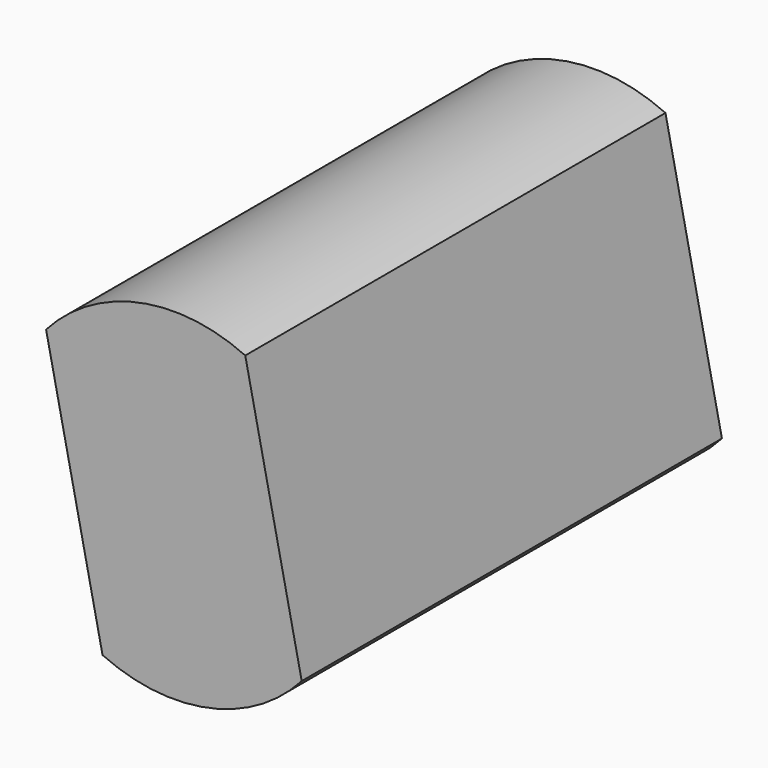
from build123d import *

# Parameters (mm, degrees)
F2_DEPTH = 8


# Not quite as in the source:
# - the program builds the solid bodies; features that only make, move or delete a surface that nothing else refers to are left out


with BuildPart() as f2:
    # F0 (on Front) → F2 (new body)
    with BuildSketch(Plane.XZ):
        with BuildLine():
            Line((1.9466441938, -1.7235360115), (1.0869146527, 2.3619095109))
            ThreePointArc((1.0869146527, 2.3619095109), (-0.5354100318, 2.5442751616), (-1.9466441938, 1.7235360115))
            Line((-1.9466441938, 1.7235360115), (-1.0869146527, -2.3619095109))
            ThreePointArc((-1.0869146527, -2.3619095109), (0.5354100318, -2.5442751616), (1.9466441938, -1.7235360115))
        make_face()
    extrude(amount=F2_DEPTH)


solid = f2.part
